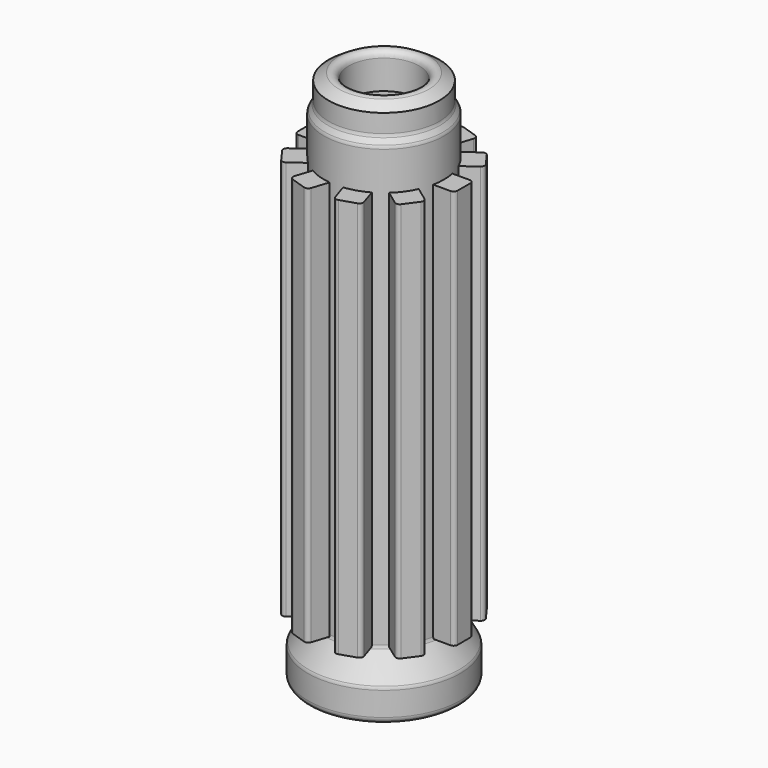
from build123d import *

# Parameters (mm, degrees)
F2_R            = 1.6
F5_END_RADIUS   = 15
F4_W            = 6
F4_H            = 100
F5_REACH        = 139.2222902753
F5_COPIES_COUNT = 10
F6_R            = 1
F6_2_R          = 1
F6_3_R          = 1
F6_4_R          = 1
F6_5_R          = 1
F6_6_R          = 1
F6_7_R          = 1
F6_8_R          = 1
F6_9_R          = 1
F6_10_R         = 1


# Not quite as in the source:
# - a feature of the source that left no trace in its solid (it failed there, or was rolled back) is left out
# - a pattern or mirror of a feature is missing from the dataset's text; its kind, count and spacing are read off the source's solid


with BuildPart() as f1:
    # F0 (on Front) → F1 (revolve)
    with BuildSketch(Plane.XZ):
        with BuildLine():
            Line((10.75, 125), (10.75, 0))
            Line((10.75, 0), (19.0414518843, 0))
            Line((19.0414518843, 0), (19.0414518843, 8))
            Line((19.0414518843, 8), (15, 15))
            Line((15, 15), (15, 125))
            Line((15, 125), (13.8452994616, 127))
            Line((13.8452994616, 127), (13.8452994616, 132))
            ThreePointArc((13.8452994616, 132), (11.3726339997, 133.5737953324), (8.812, 135))
            Line((8.812, 135), (8.812, 125))
            Line((8.812, 125), (10.75, 125))
        make_face()
    revolve(axis=Axis((0, 0, 17.9382504751), (0, 0, 1)))

    # F2
    f2_edges = [f1.edges().sort_by_distance(p)[0] for p in [
        (-8.812, 0, 135),
        (-13.845299, 0, 127),
        (-15, 0, 125),
        (-15, 0, 15),
        (-19.041452, 0, 8),
        (-19.041452, 0, 0),
    ]]
    fillet(f2_edges, radius=F2_R)


with BuildPart() as f5:
    f5_end = (Plane.XY.offset(70.0000000001) * Cylinder(F5_END_RADIUS, 567.0645927536, mode=Mode.PRIVATE)).faces().sort_by_distance((-15, 0, 70.0000000001))[0]
    # F4 (on offset) → F5 (new body, up to the whole of a round face its end follows)
    with BuildSketch(Plane.YZ.offset(20)):
        with Locations((0, 65)):
            Rectangle(F4_W, F4_H)
    f5_long = extrude(amount=-F5_REACH, mode=Mode.PRIVATE)
    add(split(f5_long, bisect_by=f5_end, keep=Keep.ALL, mode=Mode.PRIVATE).solids().sort_by_distance((20, 0, 65))[0])


with BuildPart() as f5_copies_1:
    # F5_copies: instance of F5
    add(f5.part.rotate(Axis((0, 0, 0), (0, 0, 1)), 1 * 360 / F5_COPIES_COUNT))

    # F6#2
    f6_2_edges = [f5_copies_1.edges().sort_by_distance(p)[0] for p in [
        (17.943696, 9.328654, 65),
        (14.416984, 14.182756, 65),
    ]]
    fillet(f6_2_edges, radius=F6_2_R)


with BuildPart() as f5_copies_2:
    # F5_copies: instance of F5
    add(f5.part.rotate(Axis((0, 0, 0), (0, 0, 1)), 2 * 360 / F5_COPIES_COUNT))

    # F6#3
    f6_3_edges = [f5_copies_2.edges().sort_by_distance(p)[0] for p in [
        (9.033509, 18.094079, 65),
        (3.32717, 19.948181, 65),
    ]]
    fillet(f6_3_edges, radius=F6_3_R)


with BuildPart() as f5_copies_3:
    # F5_copies: instance of F5
    add(f5.part.rotate(Axis((0, 0, 0), (0, 0, 1)), 3 * 360 / F5_COPIES_COUNT))

    # F6#4
    f6_4_edges = [f5_copies_3.edges().sort_by_distance(p)[0] for p in [
        (-3.32717, 19.948181, 65),
        (-9.033509, 18.094079, 65),
    ]]
    fillet(f6_4_edges, radius=F6_4_R)


with BuildPart() as f5_copies_4:
    # F5_copies: instance of F5
    add(f5.part.rotate(Axis((0, 0, 0), (0, 0, 1)), 4 * 360 / F5_COPIES_COUNT))

    # F6#5
    f6_5_edges = [f5_copies_4.edges().sort_by_distance(p)[0] for p in [
        (-14.416984, 14.182756, 65),
        (-17.943696, 9.328654, 65),
    ]]
    fillet(f6_5_edges, radius=F6_5_R)


with BuildPart() as f5_copies_5:
    # F5_copies: instance of F5
    add(f5.part.rotate(Axis((0, 0, 0), (0, 0, 1)), 5 * 360 / F5_COPIES_COUNT))

    # F6#6
    f6_6_edges = [f5_copies_5.edges().sort_by_distance(p)[0] for p in [
        (-20, 3, 65),
        (-20, -3, 65),
    ]]
    fillet(f6_6_edges, radius=F6_6_R)


with BuildPart() as f5_copies_6:
    # F5_copies: instance of F5
    add(f5.part.rotate(Axis((0, 0, 0), (0, 0, 1)), 6 * 360 / F5_COPIES_COUNT))

    # F6#7
    f6_7_edges = [f5_copies_6.edges().sort_by_distance(p)[0] for p in [
        (-17.943696, -9.328654, 65),
        (-14.416984, -14.182756, 65),
    ]]
    fillet(f6_7_edges, radius=F6_7_R)


with BuildPart() as f5_copies_7:
    # F5_copies: instance of F5
    add(f5.part.rotate(Axis((0, 0, 0), (0, 0, 1)), 7 * 360 / F5_COPIES_COUNT))

    # F6#8
    f6_8_edges = [f5_copies_7.edges().sort_by_distance(p)[0] for p in [
        (-9.033509, -18.094079, 65),
        (-3.32717, -19.948181, 65),
    ]]
    fillet(f6_8_edges, radius=F6_8_R)


with BuildPart() as f5_copies_8:
    # F5_copies: instance of F5
    add(f5.part.rotate(Axis((0, 0, 0), (0, 0, 1)), 8 * 360 / F5_COPIES_COUNT))

    # F6#9
    f6_9_edges = [f5_copies_8.edges().sort_by_distance(p)[0] for p in [
        (3.32717, -19.948181, 65),
        (9.033509, -18.094079, 65),
    ]]
    fillet(f6_9_edges, radius=F6_9_R)


with BuildPart() as f5_copies_9:
    # F5_copies: instance of F5
    add(f5.part.rotate(Axis((0, 0, 0), (0, 0, 1)), 9 * 360 / F5_COPIES_COUNT))

    # F6#10
    f6_10_edges = [f5_copies_9.edges().sort_by_distance(p)[0] for p in [
        (14.416984, -14.182756, 65),
        (17.943696, -9.328654, 65),
    ]]
    fillet(f6_10_edges, radius=F6_10_R)


with BuildPart() as f5_1:
    add(f5.part)

    # F6
    f6_edges = [f5_1.edges().sort_by_distance(p)[0] for p in [
        (20, -3, 65),
        (20, 3, 65),
    ]]
    fillet(f6_edges, radius=F6_R)


solid = Compound([f1.part, f5_copies_1.part, f5_copies_2.part, f5_copies_3.part, f5_copies_4.part, f5_copies_5.part, f5_copies_6.part, f5_copies_7.part, f5_copies_8.part, f5_copies_9.part, f5_1.part])
